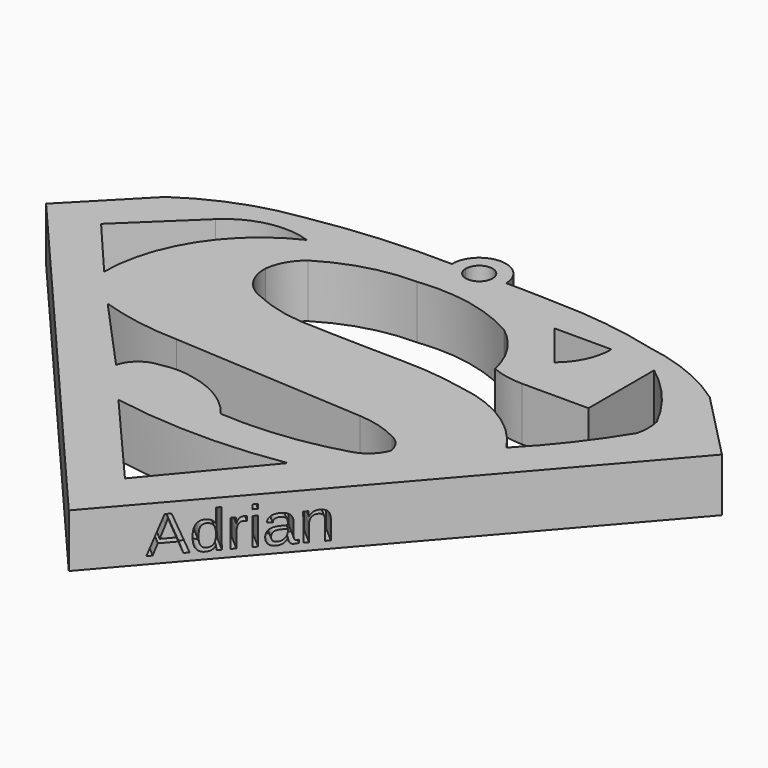
from build123d import *

# Parameters (mm, degrees)
F1_DEPTH     = 5
F2_TEXT_SIZE = 4.8596990382
F3_DEPTH     = 2


# Not quite as in the source:
# - Text() gives the source's letters only with a copy of the font that has no kerning and outlines rounded to 1/6400 em; it was checked with that copy


with BuildPart() as f1:
    # F0 (on Top) → F1 (new body)
    with BuildSketch(Plane.XY):
        with BuildLine():
            Line((7.3919766583, 44.0557971597), (1.2666468974, 37.7875715494))
            Line((1.2666468974, 37.7875715494), (32.8947368421, 0.9089741687))
            Line((32.8947368421, 0.9089741687), (64.6540150046, 37.638604641))
            Line((64.6540150046, 37.638604641), (58.2880862057, 44.1708602011))
            ThreePointArc((58.2880862057, 44.1708602011), (54.3210726028, 46.346668622), (49.9593727291, 47.5495457649))
            ThreePointArc((49.9593727291, 47.5495457649), (45.0529442092, 48.5121015436), (40.065202862, 48.8613732159))
            ThreePointArc((40.065202862, 48.8613732159), (37.7304725249, 48.9402082881), (35.3945623882, 48.9667516377))
            ThreePointArc((35.3945623882, 48.9667516377), (35.3946932283, 48.9519850485), (35.3947368421, 48.937217944))
            ThreePointArc((35.3947368421, 48.937217944), (32.92855714, 46.437446717), (30.3956518921, 48.869583538))
            ThreePointArc((30.3956518921, 48.869583538), (23.8424748783, 48.7041827946), (17.3400919884, 47.8732176125))
            ThreePointArc((17.3400919884, 47.8732176125), (12.1375338454, 46.5599747012), (7.3919766583, 44.0557971597))
        make_face()
        with BuildLine():
            Line((32.9362899065, 7.4282735586), (24.7843433172, 16.8565288186))
            ThreePointArc((24.7843433172, 16.8565288186), (32.7480685443, 16.1432721808), (40.719602257, 16.7631953955))
            Line((40.719602257, 16.7631953955), (32.9362899065, 7.4282735586))
        make_face(mode=Mode.SUBTRACT)
        with BuildLine():
            Line((21.1969863746, 21.0609231144), (14.6789392456, 28.2322764397))
            ThreePointArc((14.6789392456, 28.2322764397), (18.3461220616, 27.3372205828), (22.1045967191, 26.9861891866))
            Line((22.1045967191, 26.9861891866), (40.1855669916, 25.8926842362))
            ThreePointArc((40.1855669916, 25.8926842362), (42.1620748775, 25.5618486686), (44.0255440772, 24.8246118426))
            ThreePointArc((44.0255440772, 24.8246118426), (44.9460556292, 24.0754479323), (45.3733541071, 22.9681972414))
            ThreePointArc((45.3733541071, 22.9681972414), (44.555026805, 21.7860299384), (43.3134958148, 21.0609231144))
            ThreePointArc((43.3134958148, 21.0609231144), (37.7248157002, 19.9203019351), (32.0224277675, 19.7894051671))
            ThreePointArc((32.0224277675, 19.7894051671), (29.6444320584, 21.9381514557), (26.6459193701, 23.0699181557))
            ThreePointArc((26.6459193701, 23.0699181557), (25.1890290839, 23.2486524013), (23.7321387976, 23.0699181557))
            ThreePointArc((23.7321387976, 23.0699181557), (22.1392776506, 22.4758979511), (21.1969863746, 21.0609231144))
        make_face(mode=Mode.SUBTRACT)
        with BuildLine():
            ThreePointArc((19.7429414839, 45.2129207551), (13.6207727272, 39.8481403339), (11.2967044115, 32.0468246937))
            Line((11.2967044115, 32.0468246937), (6.4003244042, 37.8043539822))
            Line((6.4003244042, 37.8043539822), (12.4664995819, 43.6176285148))
            ThreePointArc((12.4664995819, 43.6176285148), (15.8804033867, 45.4384292899), (19.7429414839, 45.2129207551))
        make_face(mode=Mode.SUBTRACT)
        with BuildLine():
            Line((52.4514578283, 37.2771285474), (52.4514578283, 44.9585802853))
            ThreePointArc((52.4514578283, 44.9585802853), (55.4258541853, 42.1479304161), (57.6875321567, 38.7374173857))
            ThreePointArc((57.6875321567, 38.7374173857), (57.825861918, 37.5754373152), (57.6875321567, 36.4134572446))
            ThreePointArc((57.6875321567, 36.4134572446), (54.8977234657, 32.3639091345), (51.6651682556, 28.658175841))
            ThreePointArc((51.6651682556, 28.658175841), (48.0253853269, 32.2372601855), (43.2276688516, 33.9807569981))
            ThreePointArc((43.2276688516, 33.9807569981), (40.2919870848, 34.4533078111), (37.3235940933, 34.6270166337))
            ThreePointArc((37.3235940933, 34.6270166337), (32.3630009332, 34.7104740261), (27.4042375386, 34.8689518869))
            ThreePointArc((27.4042375386, 34.8689518869), (24.9573843441, 35.2868167163), (22.6260125637, 36.1391119659))
            ThreePointArc((22.6260125637, 36.1391119659), (20.8222503627, 37.5759658042), (20.2066581696, 39.798386395))
            ThreePointArc((20.2066581696, 39.798386395), (20.730686564, 41.427957292), (21.8397211283, 42.7318550646))
            ThreePointArc((21.8397211283, 42.7318550646), (25.8353051393, 44.4946984912), (30.1631521434, 45.0795479119))
            ThreePointArc((30.1631521434, 45.0795479119), (35.1749361328, 44.8767297326), (39.870813489, 43.1138202548))
            ThreePointArc((39.870813489, 43.1138202548), (42.0178475199, 40.7985600889), (43.2276688516, 37.8819666803))
            ThreePointArc((43.2276688516, 37.8819666803), (44.6944032233, 37.4298501723), (46.2216213346, 37.2771285474))
            Line((46.2216213346, 37.2771285474), (52.4514578283, 37.2771285474))
        make_face(mode=Mode.SUBTRACT)
        with BuildLine():
            Line((45.9796823561, 41.3900315762), (42.6228307188, 45.5936603248))
            Line((42.6228307188, 45.5936603248), (47.9454100132, 45.5936603248))
            ThreePointArc((47.9454100132, 45.5936603248), (47.4445519598, 43.266447339), (45.9796823561, 41.3900315762))
        make_face(mode=Mode.SUBTRACT)
        with BuildLine():
            ThreePointArc((35.3945623882, 48.9667516377), (32.8461513811, 51.43674579), (30.3956518921, 48.869583538))
            ThreePointArc((30.3956518921, 48.869583538), (30.5423349236, 48.8656455412), (30.689008598, 48.8613732159))
            ThreePointArc((30.689008598, 48.8613732159), (31.1671056556, 48.8817790665), (31.6452912767, 48.8999918908))
            ThreePointArc((31.6452912767, 48.8999918908), (32.8649961237, 50.1868640898), (34.1445387246, 48.9594722603))
            ThreePointArc((34.1445387246, 48.9594722603), (34.7695396543, 48.9649840654), (35.3945623882, 48.9667516377))
        make_face()
        with BuildLine():
            ThreePointArc((30.689008598, 48.8613732159), (30.5423349236, 48.8656455412), (30.3956518921, 48.869583538))
            ThreePointArc((30.3956518921, 48.869583538), (32.92855714, 46.437446717), (35.3947368421, 48.937217944))
            ThreePointArc((35.3947368421, 48.937217944), (35.3946932283, 48.9519850485), (35.3945623882, 48.9667516377))
            ThreePointArc((35.3945623882, 48.9667516377), (34.7695396543, 48.9649840654), (34.1445387246, 48.9594722603))
            ThreePointArc((34.1445387246, 48.9594722603), (34.1446873117, 48.9483455431), (34.1447368421, 48.937217944))
            ThreePointArc((34.1447368421, 48.937217944), (32.913351933, 47.6873565603), (31.6452912767, 48.8999918908))
            ThreePointArc((31.6452912767, 48.8999918908), (31.1671056556, 48.8817790665), (30.689008598, 48.8613732159))
        make_face()
    extrude(amount=F1_DEPTH)

    # F2 (on face) → F3 (cut)
    with BuildSketch(Plane(origin=(18.3723616526, -15.8861642964, 0), x_dir=(0.6540707669, 0.7564333625, 0), z_dir=(0.7564333625, -0.6540707669, 0))):
        with Locations((27.9562342912, 0.6818890979)):
            Text('Adrian', F2_TEXT_SIZE, font='Arimo', text_align=(TextAlign.LEFT, TextAlign.BOTTOM))
    extrude(amount=-F3_DEPTH, mode=Mode.SUBTRACT)


solid = f1.part
